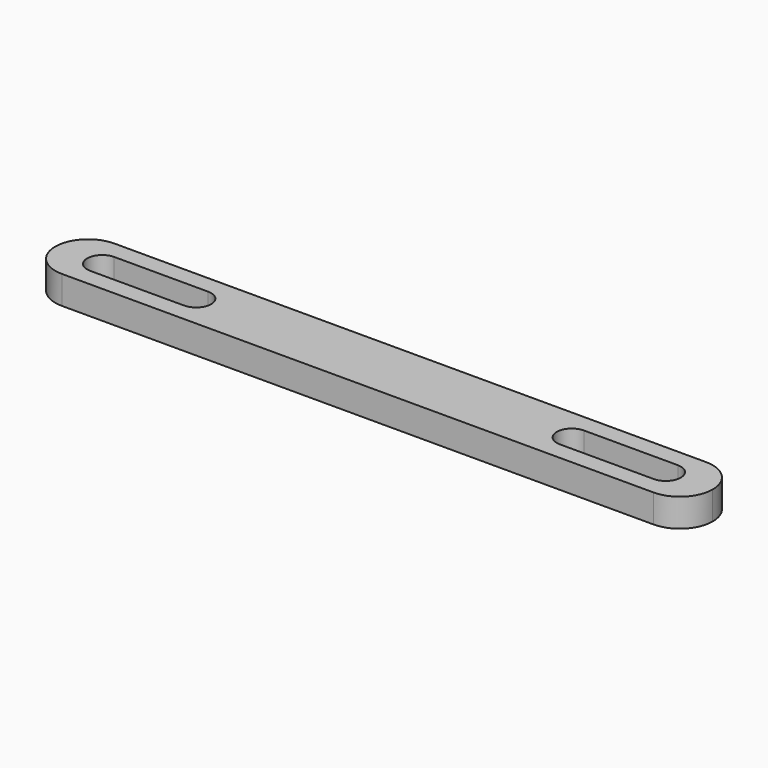
from build123d import *

# Parameters (mm, degrees)
F0_W     = 70
F0_H     = 7
F1_DEPTH = 3
F2_R     = 3.49999


# Not quite as in the source:
# - a fillet or chamfer is up to 0.001 mm smaller than in the source, because OpenCascade refuses the exact size


with BuildPart() as f1:
    # F0 (on Top) → F1 (new body)
    with BuildSketch(Plane.XY):
        Rectangle(F0_W, F0_H)
        with BuildLine():
            Line((-20, -1.6), (-30, -1.6))
            ThreePointArc((-30, -1.6), (-31.6, 0), (-30, 1.6))
            Line((-30, 1.6), (-20, 1.6))
            ThreePointArc((-20, 1.6), (-18.4, 0), (-20, -1.6))
        make_face(mode=Mode.SUBTRACT)
        with BuildLine():
            Line((20, 1.6), (30, 1.6))
            ThreePointArc((30, 1.6), (31.6, 0), (30, -1.6))
            Line((30, -1.6), (20, -1.6))
            ThreePointArc((20, -1.6), (18.4, 0), (20, 1.6))
        make_face(mode=Mode.SUBTRACT)
    extrude(amount=F1_DEPTH)

    # F2 (radius 3.5 in the source; OpenCascade refuses exactly that, so slightly less here)
    f2_edges = [f1.edges().sort_by_distance(p)[0] for p in [
        (-35, 3.5, 1.5),
        (-35, -3.5, 1.5),
        (35, 3.5, 1.5),
        (35, -3.5, 1.5),
    ]]
    fillet(f2_edges, radius=F2_R)


solid = f1.part
